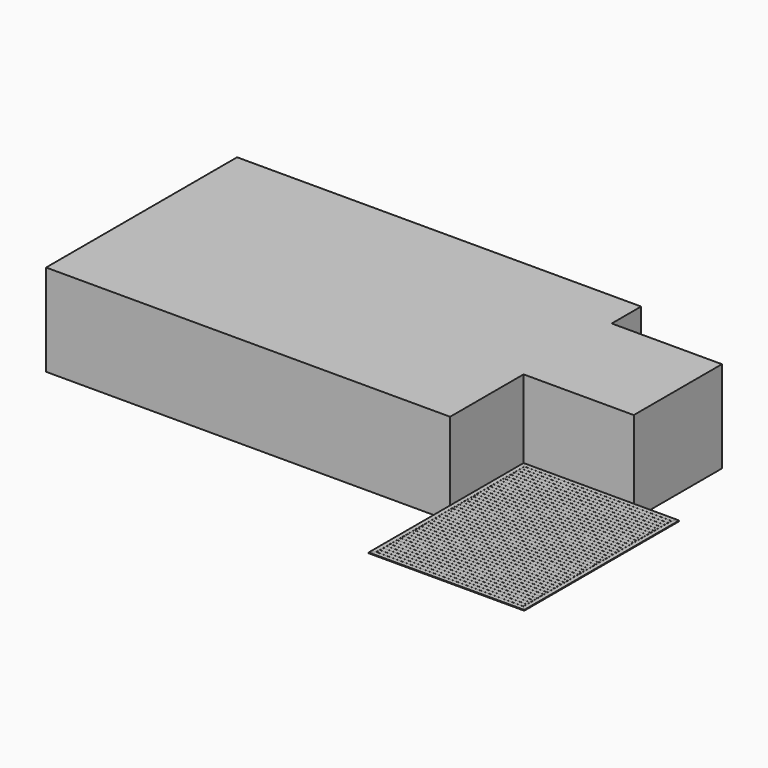
from build123d import *

# Parameters (mm, degrees)
F1_DEPTH  = 3048
F4_DEPTH  = 25.4
F6_DEPTH  = 25.4
F7_W      = 4876.8
F7_H      = 139.7
F8_DEPTH  = 25.4
F10_DEPTH = 25.4
F12_DEPTH = 25.4


with BuildPart() as f1:
    # F0 (on Top) → F1 (new body)
    with BuildSketch(Plane.XY):
        Polygon((0, 4876.8), (-13411.2, 4876.8), (-13411.2, -3048), (0, -3048), (0, 0), (3657.6, 0), (3657.6, 3657.6), (0, 3657.6), align=None)
    extrude(amount=F1_DEPTH)

    # F3 (on offset) → F4 (join)
    with BuildSketch(Plane(origin=(0, 0, 431.8), x_dir=(1, 0, 0), z_dir=(0, 0, -1))):
        Polygon((139.7, 139.7), (0, 0), (5162.55, 0), (5022.85, 139.7), align=None)
    extrude(amount=-F4_DEPTH)

    # F5 (on offset) → F6 (join)
    with BuildSketch(Plane(origin=(0, 0, 431.8), x_dir=(1, 0, 0), z_dir=(0, 0, -1))):
        Polygon((0, 6426.2359210245), (0, 0.0359210245), (139.7, 139.7359210245), (139.7, 6286.5359210245), align=None)
    extrude(amount=-F6_DEPTH)


with BuildPart() as f8:
    # F7 (on offset) → F8 (new body)
    with BuildSketch(Plane(origin=(0, 0, 431.8), x_dir=(1, 0, 0), z_dir=(0, 0, -1))):
        with Locations((2581.275, 212.725)):
            Rectangle(F7_W, F7_H)
    extrude(amount=-F8_DEPTH)


with BuildPart() as f8b:
    # F7 (on offset) → F8, piece 2 (new body)
    with BuildSketch(Plane(origin=(0, 0, 431.8), x_dir=(1, 0, 0), z_dir=(0, 0, -1))):
        with Locations((2581.275, 355.6)):
            Rectangle(F7_W, F7_H)
    extrude(amount=-F8_DEPTH)


with BuildPart() as f8c:
    # F7 (on offset) → F8, piece 3 (new body)
    with BuildSketch(Plane(origin=(0, 0, 431.8), x_dir=(1, 0, 0), z_dir=(0, 0, -1))):
        with Locations((2581.275, 498.475)):
            Rectangle(F7_W, F7_H)
    extrude(amount=-F8_DEPTH)


with BuildPart() as f8d:
    # F7 (on offset) → F8, piece 4 (new body)
    with BuildSketch(Plane(origin=(0, 0, 431.8), x_dir=(1, 0, 0), z_dir=(0, 0, -1))):
        with Locations((2581.275, 641.35)):
            Rectangle(F7_W, F7_H)
    extrude(amount=-F8_DEPTH)


with BuildPart() as f8e:
    # F7 (on offset) → F8, piece 5 (new body)
    with BuildSketch(Plane(origin=(0, 0, 431.8), x_dir=(1, 0, 0), z_dir=(0, 0, -1))):
        with Locations((2581.275, 784.225)):
            Rectangle(F7_W, F7_H)
    extrude(amount=-F8_DEPTH)


with BuildPart() as f8f:
    # F7 (on offset) → F8, piece 6 (new body)
    with BuildSketch(Plane(origin=(0, 0, 431.8), x_dir=(1, 0, 0), z_dir=(0, 0, -1))):
        with Locations((2581.275, 927.1)):
            Rectangle(F7_W, F7_H)
    extrude(amount=-F8_DEPTH)


with BuildPart() as f8g:
    # F7 (on offset) → F8, piece 7 (new body)
    with BuildSketch(Plane(origin=(0, 0, 431.8), x_dir=(1, 0, 0), z_dir=(0, 0, -1))):
        with Locations((2581.275, 1069.975)):
            Rectangle(F7_W, F7_H)
    extrude(amount=-F8_DEPTH)


with BuildPart() as f8h:
    # F7 (on offset) → F8, piece 8 (new body)
    with BuildSketch(Plane(origin=(0, 0, 431.8), x_dir=(1, 0, 0), z_dir=(0, 0, -1))):
        with Locations((2581.275, 1212.85)):
            Rectangle(F7_W, F7_H)
    extrude(amount=-F8_DEPTH)


with BuildPart() as f8i:
    # F7 (on offset) → F8, piece 9 (new body)
    with BuildSketch(Plane(origin=(0, 0, 431.8), x_dir=(1, 0, 0), z_dir=(0, 0, -1))):
        with Locations((2581.275, 1355.725)):
            Rectangle(F7_W, F7_H)
    extrude(amount=-F8_DEPTH)


with BuildPart() as f8j:
    # F7 (on offset) → F8, piece 10 (new body)
    with BuildSketch(Plane(origin=(0, 0, 431.8), x_dir=(1, 0, 0), z_dir=(0, 0, -1))):
        with Locations((2581.275, 1498.6)):
            Rectangle(F7_W, F7_H)
    extrude(amount=-F8_DEPTH)


with BuildPart() as f8k:
    # F7 (on offset) → F8, piece 11 (new body)
    with BuildSketch(Plane(origin=(0, 0, 431.8), x_dir=(1, 0, 0), z_dir=(0, 0, -1))):
        with Locations((2581.275, 1641.475)):
            Rectangle(F7_W, F7_H)
    extrude(amount=-F8_DEPTH)


with BuildPart() as f8l:
    # F7 (on offset) → F8, piece 12 (new body)
    with BuildSketch(Plane(origin=(0, 0, 431.8), x_dir=(1, 0, 0), z_dir=(0, 0, -1))):
        with Locations((2581.275, 1784.35)):
            Rectangle(F7_W, F7_H)
    extrude(amount=-F8_DEPTH)


with BuildPart() as f8m:
    # F7 (on offset) → F8, piece 13 (new body)
    with BuildSketch(Plane(origin=(0, 0, 431.8), x_dir=(1, 0, 0), z_dir=(0, 0, -1))):
        with Locations((2581.275, 1927.225)):
            Rectangle(F7_W, F7_H)
    extrude(amount=-F8_DEPTH)


with BuildPart() as f8n:
    # F7 (on offset) → F8, piece 14 (new body)
    with BuildSketch(Plane(origin=(0, 0, 431.8), x_dir=(1, 0, 0), z_dir=(0, 0, -1))):
        with Locations((2581.275, 2070.1)):
            Rectangle(F7_W, F7_H)
    extrude(amount=-F8_DEPTH)


with BuildPart() as f8o:
    # F7 (on offset) → F8, piece 15 (new body)
    with BuildSketch(Plane(origin=(0, 0, 431.8), x_dir=(1, 0, 0), z_dir=(0, 0, -1))):
        with Locations((2581.275, 2212.975)):
            Rectangle(F7_W, F7_H)
    extrude(amount=-F8_DEPTH)


with BuildPart() as f8p:
    # F7 (on offset) → F8, piece 16 (new body)
    with BuildSketch(Plane(origin=(0, 0, 431.8), x_dir=(1, 0, 0), z_dir=(0, 0, -1))):
        with Locations((2581.275, 2355.85)):
            Rectangle(F7_W, F7_H)
    extrude(amount=-F8_DEPTH)


with BuildPart() as f8q:
    # F7 (on offset) → F8, piece 17 (new body)
    with BuildSketch(Plane(origin=(0, 0, 431.8), x_dir=(1, 0, 0), z_dir=(0, 0, -1))):
        with Locations((2581.275, 2498.725)):
            Rectangle(F7_W, F7_H)
    extrude(amount=-F8_DEPTH)


with BuildPart() as f8r:
    # F7 (on offset) → F8, piece 18 (new body)
    with BuildSketch(Plane(origin=(0, 0, 431.8), x_dir=(1, 0, 0), z_dir=(0, 0, -1))):
        with Locations((2581.275, 2641.6)):
            Rectangle(F7_W, F7_H)
    extrude(amount=-F8_DEPTH)


with BuildPart() as f8s:
    # F7 (on offset) → F8, piece 19 (new body)
    with BuildSketch(Plane(origin=(0, 0, 431.8), x_dir=(1, 0, 0), z_dir=(0, 0, -1))):
        with Locations((2581.275, 2784.475)):
            Rectangle(F7_W, F7_H)
    extrude(amount=-F8_DEPTH)


with BuildPart() as f8t:
    # F7 (on offset) → F8, piece 20 (new body)
    with BuildSketch(Plane(origin=(0, 0, 431.8), x_dir=(1, 0, 0), z_dir=(0, 0, -1))):
        with Locations((2581.275, 2927.35)):
            Rectangle(F7_W, F7_H)
    extrude(amount=-F8_DEPTH)


with BuildPart() as f8u:
    # F7 (on offset) → F8, piece 21 (new body)
    with BuildSketch(Plane(origin=(0, 0, 431.8), x_dir=(1, 0, 0), z_dir=(0, 0, -1))):
        with Locations((2581.275, 3070.225)):
            Rectangle(F7_W, F7_H)
    extrude(amount=-F8_DEPTH)


with BuildPart() as f8v:
    # F7 (on offset) → F8, piece 22 (new body)
    with BuildSketch(Plane(origin=(0, 0, 431.8), x_dir=(1, 0, 0), z_dir=(0, 0, -1))):
        with Locations((2581.275, 3213.1)):
            Rectangle(F7_W, F7_H)
    extrude(amount=-F8_DEPTH)


with BuildPart() as f8w:
    # F7 (on offset) → F8, piece 23 (new body)
    with BuildSketch(Plane(origin=(0, 0, 431.8), x_dir=(1, 0, 0), z_dir=(0, 0, -1))):
        with Locations((2581.275, 3355.975)):
            Rectangle(F7_W, F7_H)
    extrude(amount=-F8_DEPTH)


with BuildPart() as f8x:
    # F7 (on offset) → F8, piece 24 (new body)
    with BuildSketch(Plane(origin=(0, 0, 431.8), x_dir=(1, 0, 0), z_dir=(0, 0, -1))):
        with Locations((2581.275, 3498.85)):
            Rectangle(F7_W, F7_H)
    extrude(amount=-F8_DEPTH)


with BuildPart() as f8y:
    # F7 (on offset) → F8, piece 25 (new body)
    with BuildSketch(Plane(origin=(0, 0, 431.8), x_dir=(1, 0, 0), z_dir=(0, 0, -1))):
        with Locations((2581.275, 3641.725)):
            Rectangle(F7_W, F7_H)
    extrude(amount=-F8_DEPTH)


with BuildPart() as f8z:
    # F7 (on offset) → F8, piece 26 (new body)
    with BuildSketch(Plane(origin=(0, 0, 431.8), x_dir=(1, 0, 0), z_dir=(0, 0, -1))):
        with Locations((2581.275, 3784.6)):
            Rectangle(F7_W, F7_H)
    extrude(amount=-F8_DEPTH)


with BuildPart() as f8ba:
    # F7 (on offset) → F8, piece 27 (new body)
    with BuildSketch(Plane(origin=(0, 0, 431.8), x_dir=(1, 0, 0), z_dir=(0, 0, -1))):
        with Locations((2581.275, 3927.475)):
            Rectangle(F7_W, F7_H)
    extrude(amount=-F8_DEPTH)


with BuildPart() as f8bb:
    # F7 (on offset) → F8, piece 28 (new body)
    with BuildSketch(Plane(origin=(0, 0, 431.8), x_dir=(1, 0, 0), z_dir=(0, 0, -1))):
        with Locations((2581.275, 4070.35)):
            Rectangle(F7_W, F7_H)
    extrude(amount=-F8_DEPTH)


with BuildPart() as f8bc:
    # F7 (on offset) → F8, piece 29 (new body)
    with BuildSketch(Plane(origin=(0, 0, 431.8), x_dir=(1, 0, 0), z_dir=(0, 0, -1))):
        with Locations((2581.275, 4213.225)):
            Rectangle(F7_W, F7_H)
    extrude(amount=-F8_DEPTH)


with BuildPart() as f8bd:
    # F7 (on offset) → F8, piece 30 (new body)
    with BuildSketch(Plane(origin=(0, 0, 431.8), x_dir=(1, 0, 0), z_dir=(0, 0, -1))):
        with Locations((2581.275, 4356.1)):
            Rectangle(F7_W, F7_H)
    extrude(amount=-F8_DEPTH)


with BuildPart() as f8be:
    # F7 (on offset) → F8, piece 31 (new body)
    with BuildSketch(Plane(origin=(0, 0, 431.8), x_dir=(1, 0, 0), z_dir=(0, 0, -1))):
        with Locations((2581.275, 4498.975)):
            Rectangle(F7_W, F7_H)
    extrude(amount=-F8_DEPTH)


with BuildPart() as f8bf:
    # F7 (on offset) → F8, piece 32 (new body)
    with BuildSketch(Plane(origin=(0, 0, 431.8), x_dir=(1, 0, 0), z_dir=(0, 0, -1))):
        with Locations((2581.275, 4641.85)):
            Rectangle(F7_W, F7_H)
    extrude(amount=-F8_DEPTH)


with BuildPart() as f8bg:
    # F7 (on offset) → F8, piece 33 (new body)
    with BuildSketch(Plane(origin=(0, 0, 431.8), x_dir=(1, 0, 0), z_dir=(0, 0, -1))):
        with Locations((2581.275, 4784.725)):
            Rectangle(F7_W, F7_H)
    extrude(amount=-F8_DEPTH)


with BuildPart() as f8bh:
    # F7 (on offset) → F8, piece 34 (new body)
    with BuildSketch(Plane(origin=(0, 0, 431.8), x_dir=(1, 0, 0), z_dir=(0, 0, -1))):
        with Locations((2581.275, 4927.6)):
            Rectangle(F7_W, F7_H)
    extrude(amount=-F8_DEPTH)


with BuildPart() as f8bi:
    # F7 (on offset) → F8, piece 35 (new body)
    with BuildSketch(Plane(origin=(0, 0, 431.8), x_dir=(1, 0, 0), z_dir=(0, 0, -1))):
        with Locations((2581.275, 5070.475)):
            Rectangle(F7_W, F7_H)
    extrude(amount=-F8_DEPTH)


with BuildPart() as f8bj:
    # F7 (on offset) → F8, piece 36 (new body)
    with BuildSketch(Plane(origin=(0, 0, 431.8), x_dir=(1, 0, 0), z_dir=(0, 0, -1))):
        with Locations((2581.275, 5213.35)):
            Rectangle(F7_W, F7_H)
    extrude(amount=-F8_DEPTH)


with BuildPart() as f8bk:
    # F7 (on offset) → F8, piece 37 (new body)
    with BuildSketch(Plane(origin=(0, 0, 431.8), x_dir=(1, 0, 0), z_dir=(0, 0, -1))):
        with Locations((2581.275, 5356.225)):
            Rectangle(F7_W, F7_H)
    extrude(amount=-F8_DEPTH)


with BuildPart() as f8bl:
    # F7 (on offset) → F8, piece 38 (new body)
    with BuildSketch(Plane(origin=(0, 0, 431.8), x_dir=(1, 0, 0), z_dir=(0, 0, -1))):
        with Locations((2581.275, 5499.1)):
            Rectangle(F7_W, F7_H)
    extrude(amount=-F8_DEPTH)


with BuildPart() as f8bm:
    # F7 (on offset) → F8, piece 39 (new body)
    with BuildSketch(Plane(origin=(0, 0, 431.8), x_dir=(1, 0, 0), z_dir=(0, 0, -1))):
        with Locations((2581.275, 5641.975)):
            Rectangle(F7_W, F7_H)
    extrude(amount=-F8_DEPTH)


with BuildPart() as f8bn:
    # F7 (on offset) → F8, piece 40 (new body)
    with BuildSketch(Plane(origin=(0, 0, 431.8), x_dir=(1, 0, 0), z_dir=(0, 0, -1))):
        with Locations((2581.275, 5784.85)):
            Rectangle(F7_W, F7_H)
    extrude(amount=-F8_DEPTH)


with BuildPart() as f8bo:
    # F7 (on offset) → F8, piece 41 (new body)
    with BuildSketch(Plane(origin=(0, 0, 431.8), x_dir=(1, 0, 0), z_dir=(0, 0, -1))):
        with Locations((2581.275, 5927.725)):
            Rectangle(F7_W, F7_H)
    extrude(amount=-F8_DEPTH)


with BuildPart() as f8bp:
    # F7 (on offset) → F8, piece 42 (new body)
    with BuildSketch(Plane(origin=(0, 0, 431.8), x_dir=(1, 0, 0), z_dir=(0, 0, -1))):
        with Locations((2581.275, 6070.6)):
            Rectangle(F7_W, F7_H)
    extrude(amount=-F8_DEPTH)


with BuildPart() as f8bq:
    # F7 (on offset) → F8, piece 43 (new body)
    with BuildSketch(Plane(origin=(0, 0, 431.8), x_dir=(1, 0, 0), z_dir=(0, 0, -1))):
        with Locations((2581.275, 6213.475)):
            Rectangle(F7_W, F7_H)
    extrude(amount=-F8_DEPTH)


with BuildPart() as f10:
    # F9 (on offset) → F10 (new body)
    with BuildSketch(Plane(origin=(0, 0, 431.8), x_dir=(1, 0, 0), z_dir=(0, 0, -1))):
        Polygon((5022.85, 139.7359210245), (5162.55, 0.0359210245), (5162.55, 6426.2), (5022.85, 6286.5), align=None)
    extrude(amount=-F10_DEPTH)


with BuildPart() as f12:
    # F11 (on offset) → F12 (new body)
    with BuildSketch(Plane(origin=(0, 0, 431.8), x_dir=(1, 0, 0), z_dir=(0, 0, -1))):
        Polygon((5162.5140789755, 6426.2), (0.071842049, 6426.2), (139.771842049, 6286.5), (5022.8140789755, 6286.5), align=None)
    extrude(amount=-F12_DEPTH)


solid = Compound([f1.part, f8.part, f8b.part, f8c.part, f8d.part, f8e.part, f8f.part, f8g.part, f8h.part, f8i.part, f8j.part, f8k.part, f8l.part, f8m.part, f8n.part, f8o.part, f8p.part, f8q.part, f8r.part, f8s.part, f8t.part, f8u.part, f8v.part, f8w.part, f8x.part, f8y.part, f8z.part, f8ba.part, f8bb.part, f8bc.part, f8bd.part, f8be.part, f8bf.part, f8bg.part, f8bh.part, f8bi.part, f8bj.part, f8bk.part, f8bl.part, f8bm.part, f8bn.part, f8bo.part, f8bp.part, f8bq.part, f10.part, f12.part])
